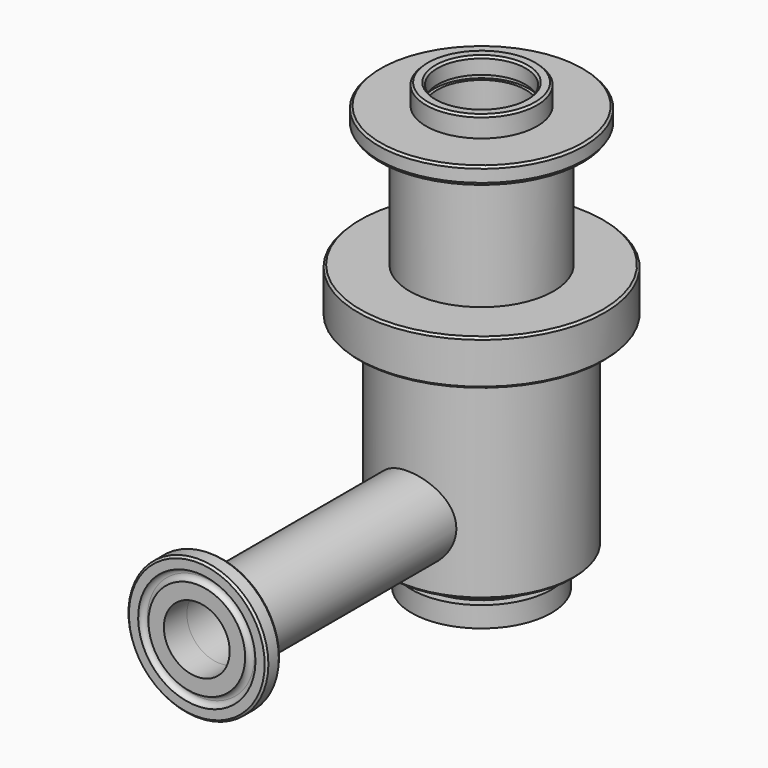
from build123d import *

# Parameters (mm, degrees)
F0_R           = 13.5
F0_R_2         = 10.75
F1_DEPTH       = 5
F2_R           = 25
F2_R_2         = 13.5
F2_R_3         = 10.75
F3_DEPTH       = 7
F4_R           = 17.5
F5_DEPTH       = 27
F6_R           = 30
F6_R_2         = 17.5
F7_DEPTH       = 11
F8_R           = 22.5
F9_DEPTH       = 49
F10_R          = 15
F11_DEPTH      = 4
F12_R          = 17
F12_R_2        = 15
F13_DEPTH      = 5
F14_R          = 11.5
F15_DEPTH      = 37
F16_R          = 10.75
F17_DEPTH      = 103.001
F18_SIZE       = 0.5
F19_SIZE2      = 2.99999
F19_SIZE       = 7.49999
F20_SIZE       = 0.5
F22_R          = 10
F23_DEPTH      = 57
F23_DEPTH_BACK = 11
F24_R          = 8
F25_DEPTH      = 71.2396442793
F26_R          = 17
F26_R_2        = 10
F26_R_3        = 8
F27_DEPTH      = 7
F28_SIZE2      = 6.99999
F28_SIZE       = 2.99999
F30_R          = 1.25
F33_R          = 11.5
F34_DEPTH      = 1.1


# Not quite as in the source:
# - a fillet or chamfer that OpenCascade refuses, or shapes differently, is made with other operations: its cross-section is extruded or revolved along the edge and cut away or added
# - a fillet or chamfer is up to 0.001 mm smaller than in the source, because OpenCascade refuses the exact size


with BuildPart() as f1:
    # F0 (on Top) → F1 (new body)
    with BuildSketch(Plane.XY):
        Circle(F0_R)
        Circle(F0_R_2, mode=Mode.SUBTRACT)
    extrude(amount=F1_DEPTH)

    # F2 (on face) → F3 (join)
    with BuildSketch(Plane(origin=(0, 0, 0), x_dir=(1, 0, 0), z_dir=(0, 0, -1))):
        Circle(F2_R)
        Circle(F2_R_2, mode=Mode.SUBTRACT)
        Circle(F2_R_2)
        Circle(F2_R_3, mode=Mode.SUBTRACT)
    extrude(amount=F3_DEPTH)

    # F4 (on face) → F5 (join)
    with BuildSketch(Plane(origin=(0, 0, -7), x_dir=(1, 0, 0), z_dir=(0, 0, -1))):
        Circle(F4_R)
    extrude(amount=F5_DEPTH)

    # F6 (on face) → F7 (join)
    with BuildSketch(Plane(origin=(0, 0, -34), x_dir=(1, 0, 0), z_dir=(0, 0, -1))):
        Circle(F6_R)
        Circle(F6_R_2, mode=Mode.SUBTRACT)
        Circle(F6_R_2)
    extrude(amount=F7_DEPTH)

    # F8 (on face) → F9 (join)
    with BuildSketch(Plane(origin=(0, 0, -45), x_dir=(1, 0, 0), z_dir=(0, 0, -1))):
        Circle(F8_R)
    extrude(amount=F9_DEPTH)

    # F10 (on face) → F11 (join)
    with BuildSketch(Plane(origin=(0, 0, -94), x_dir=(1, 0, 0), z_dir=(0, 0, -1))):
        Circle(F10_R)
    extrude(amount=F11_DEPTH)

    # F12 (on face) → F13 (join)
    with BuildSketch(Plane(origin=(0, 0, -98), x_dir=(1, 0, 0), z_dir=(0, 0, -1))):
        Circle(F12_R)
        Circle(F12_R_2, mode=Mode.SUBTRACT)
        Circle(F12_R_2)
    extrude(amount=F13_DEPTH)

    # F14 (on face) → F15 (cut)
    with BuildSketch(Plane(origin=(0, 0, -103), x_dir=(1, 0, 0), z_dir=(0, 0, -1))):
        Circle(F14_R)
    extrude(amount=-F15_DEPTH, mode=Mode.SUBTRACT)

    # F16 (on face) → F17 (cut, through all)
    with BuildSketch(Plane.XY):
        Circle(F16_R)
    extrude(amount=-F17_DEPTH, mode=Mode.SUBTRACT)

    # F18
    f18_edges = [f1.edges().sort_by_distance(p)[0] for p in [
        (-11.5, 0, -103),
        (-22.5, 0, -94),
        (-30, 0, -45),
        (-30, 0, -34),
        (-25, 0, 0),
        (-13.5, 0, 5),
        (-10.75, 0, 5),
    ]]
    chamfer(f18_edges, length=F18_SIZE)

    # F19 (size 7.5 and 3 in the source; OpenCascade refuses exactly that, so slightly less here)
    f19_edges = [f1.edges().sort_by_distance(p)[0] for p in [
        (-25, 0, -7),
    ]]
    f19_side = f1.faces().sort_by_distance((-24.292893, 0, -7))[0]
    chamfer(f19_edges, length=F19_SIZE, length2=F19_SIZE2, reference=f19_side)

    # F20
    f20_edges = [f1.edges().sort_by_distance(p)[0] for p in [
        (-25, 0, -4.00001),
    ]]
    chamfer(f20_edges, length=F20_SIZE)

    # F22 (on offset) → F23 (join, two sides)
    with BuildSketch(Plane.XZ.offset(22.5)) as f23_sk:
        with Locations((0, -79)):
            Circle(F22_R)
    extrude(amount=F23_DEPTH)
    extrude(f23_sk.sketch, amount=-F23_DEPTH_BACK)

    # F24 (on face) → F25 (cut, through all)
    with BuildSketch(Plane.XZ.offset(79.5)):
        with Locations((0, -79)):
            Circle(F24_R)
    extrude(amount=-F25_DEPTH, mode=Mode.SUBTRACT)

    # F26 (on face) → F27 (join)
    with BuildSketch(Plane.XZ.offset(79.5)):
        with Locations((0, -79)):
            Circle(F26_R)
        with Locations((0, -79)):
            Circle(F26_R_2, mode=Mode.SUBTRACT)
        with Locations((0, -79)):
            Circle(F26_R_2)
        with Locations((0, -79)):
            Circle(F26_R_3, mode=Mode.SUBTRACT)
    extrude(amount=F27_DEPTH)

    # F28 (size 3 and 7 in the source; OpenCascade refuses exactly that, so slightly less here)
    f28_edges = [f1.edges().sort_by_distance(p)[0] for p in [
        (-17, -79.5, -79),
    ]]
    f28_side = f1.faces().sort_by_distance((-17, -83, -79))[0]
    chamfer(f28_edges, length=F28_SIZE, length2=F28_SIZE2, reference=f28_side)

    # F29: chamfer of 0.5 on 2 edges, made by hand

    # F29_s1 → F29_t2 (revolve, cut)
    with BuildSketch(Plane.XY.offset(-79)):
        Polygon((17, -86), (16.5, -86.5), (17, -86.5), align=None)
    revolve(axis=Axis((0, -86.5, -79), (0, -1, 0)), mode=Mode.SUBTRACT)

    # F29_s3 → F29_t4 (revolve, cut)
    with BuildSketch(Plane.XY.offset(-79)):
        Polygon((16.6969593323, -82.3701156755), (17, -82.8296883264), (17, -82.49999), align=None)
    revolve(axis=Axis((0, -82.49999, -79), (0, -1, 0)), mode=Mode.SUBTRACT)

    # F30 (on Right) → F31 (revolve, cut)
    with BuildSketch(Plane.YZ):
        with Locations((-86.5, -66)):
            Circle(F30_R)
    revolve(axis=Axis((0, -66.6620582342, -79), (0, -1, 0)), mode=Mode.SUBTRACT)

    # F33 (on offset) → F34 (cut)
    with BuildSketch(Plane.XY.offset(1)):
        Circle(F33_R)
    extrude(amount=-F34_DEPTH, mode=Mode.SUBTRACT)


solid = f1.part
